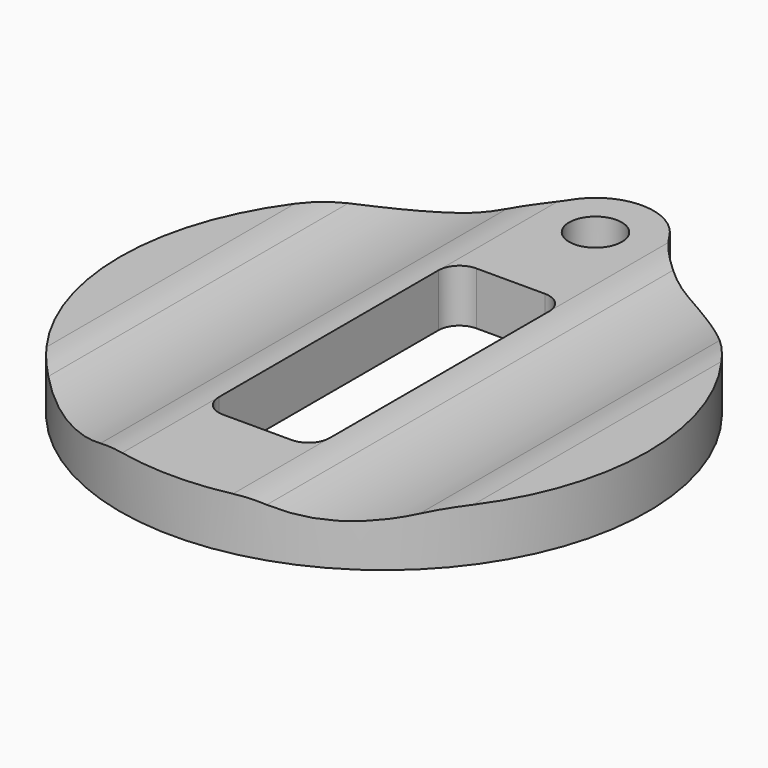
from build123d import *

# Parameters (mm, degrees)
F0_R          = 2.5
F1_DEPTH      = 2.5
F2_W          = 10.5
F2_H          = 30
F3_DEPTH      = 5.001
F5_DEPTH      = 30.5475219467
F5_DEPTH_BACK = 25.001
F6_R          = 9.99999
F7_R          = 2


# Not quite as in the source:
# - a fillet or chamfer is up to 0.001 mm smaller than in the source, because OpenCascade refuses the exact size


with BuildPart() as f1:
    # F0 (on Top) → F1 (new body, symmetric)
    with BuildSketch(Plane.XY):
        with BuildLine():
            ThreePointArc((-4.6363826998, 28.0052303576), (-7.3366406052, 24.8446324714), (-10.8006642439, 22.5465219467))
            ThreePointArc((-10.8006642439, 22.5465219467), (0, -25), (10.8006642439, 22.5465219467))
            ThreePointArc((10.8006642439, 22.5465219467), (7.3366406052, 24.8446324714), (4.6363826998, 28.0052303576))
            ThreePointArc((4.6363826998, 28.0052303576), (0, 30.5465219467), (-4.6363826998, 28.0052303576))
        make_face()
        with Locations((0, 25.0465219467)):
            Circle(F0_R, mode=Mode.SUBTRACT)
    extrude(amount=F1_DEPTH, both=True)

    # F2 (on face) → F3 (cut, through all)
    with BuildSketch(Plane.XY.offset(2.5)):
        Rectangle(F2_W, F2_H)
    extrude(amount=-F3_DEPTH, mode=Mode.SUBTRACT)

    # F4 (on Front) → F5 (cut, two sides)
    with BuildSketch(Plane.XZ) as f5_sk:
        with BuildLine():
            ThreePointArc((0, 6.579392902), (31.2333147735, 20), (0, 33.420607098))
            ThreePointArc((0, 33.420607098), (-31.2333147735, 20), (0, 6.579392902))
        make_face()
    extrude(amount=-F5_DEPTH, mode=Mode.SUBTRACT)
    extrude(f5_sk.sketch, amount=F5_DEPTH_BACK, mode=Mode.SUBTRACT)

    # F6 (radius 10 in the source; OpenCascade refuses exactly that, so slightly less here)
    f6_edges = [f1.edges().sort_by_distance(p)[0] for p in [
        (-6.733315, 0.666562, 2.5),
        (-18.733315, 0, 2.5),
        (6.733315, 0.666562, 2.5),
        (18.733315, 0, 2.5),
    ]]
    fillet(f6_edges, radius=F6_R)

    # F7
    f7_edges = [f1.edges().sort_by_distance(p)[0] for p in [
        (5.25, 15, 0),
        (5.25, -15, 0),
        (-5.25, -15, 0),
        (-5.25, 15, 0),
    ]]
    fillet(f7_edges, radius=F7_R)


solid = f1.part
